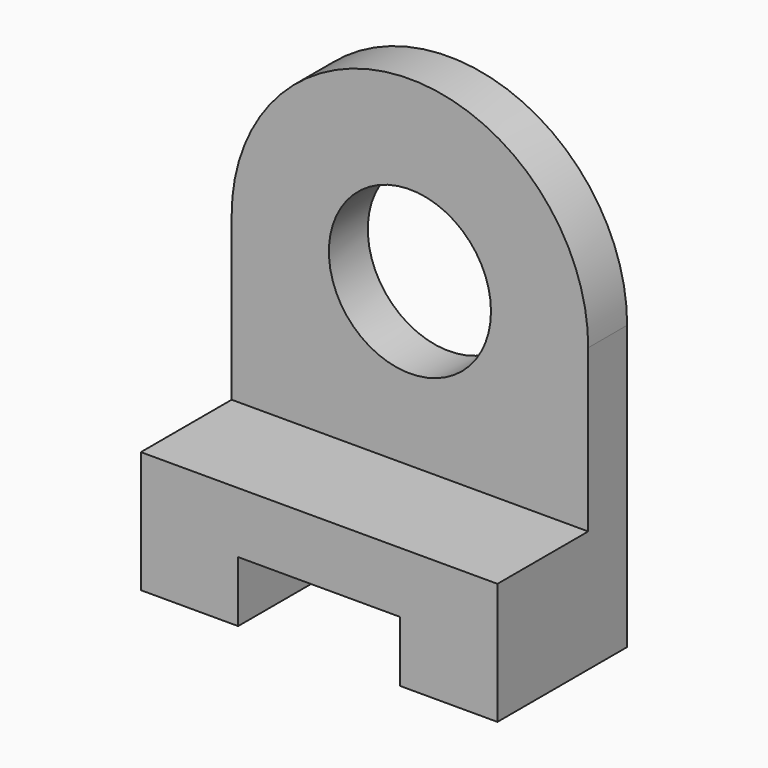
from build123d import *

# Parameters (mm, degrees)
F0_R     = 20
F1_DEPTH = 12
F3_DEPTH = 40


# Not quite as in the source:
# - the program builds the solid bodies; features that only make, move or delete a surface that nothing else refers to are left out


with BuildPart() as f1:
    # F0 (on Front) → F1 (new body)
    with BuildSketch(Plane.XZ):
        with BuildLine():
            Line((-44, 69.9118748307), (-44, 30))
            Line((-44, 30), (44, 30))
            Line((44, 30), (44, 69.9118748307))
            ThreePointArc((44, 69.9118748307), (0, 114.0000882504), (-44, 69.9118748307))
        make_face()
        with Locations((0, 70)):
            Circle(F0_R, mode=Mode.SUBTRACT)
    extrude(amount=F1_DEPTH)

    # F0 (on Front) → F3 (join)
    with BuildSketch(Plane.XZ):
        Polygon((-44, 30), (-44, 0), (-20, 0), (-20, 15), (20, 15), (20, 0), (44, 0), (44, 30), align=None)
    extrude(amount=F3_DEPTH)


solid = f1.part
